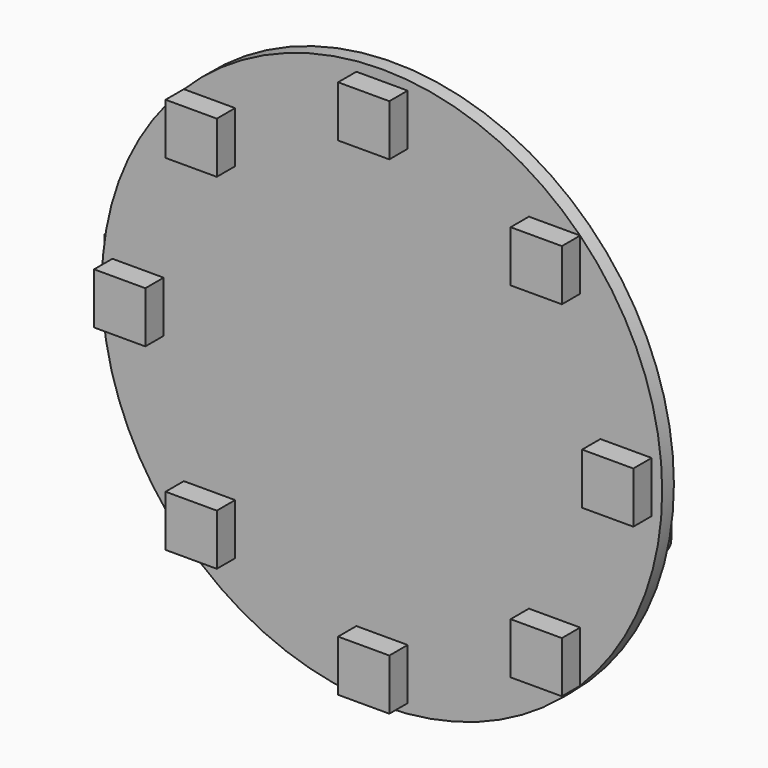
from build123d import *

# Parameters (mm, degrees)
F0_R      = 30.625
F1_DEPTH  = 1.6
F2_W      = 5.6
F2_H      = 5.6
F3_DEPTH  = 2.5
F4_W      = 16
F4_H      = 16
F5_DEPTH  = 1.6
F4_W_2    = 5.6
F4_H_2    = 5.6
F6_DEPTH  = 2.5
F4_W_3    = 3.4
F4_H_3    = 3
F4_W_4    = 1
F4_H_4    = 1.4143656492
F7_DEPTH  = 2.5
F8_DEPTH  = 3.5
F4_W_5    = 19
F4_H_5    = 8
F10_DEPTH = 4.5
F4_W_6    = 4.9
F4_H_6    = 11.6
F11_DEPTH = 0.7
F12_DEPTH = 4.3
F13_DEPTH = 3.5


# Not quite as in the source:
# - the program builds the solid bodies; features that only make, move or delete a surface that nothing else refers to are left out


with BuildPart() as f1:
    # F0 (on Front) → F1 (new body)
    with BuildSketch(Plane.XZ):
        Circle(F0_R)
    extrude(amount=F1_DEPTH)

    # F2 (on face) → F3 (join)
    with BuildSketch(Plane.XZ.offset(1.6)):
        with Locations((-26.67, 0)):
            Rectangle(F2_W, F2_H)
        with Locations((-18.8585378542, 18.8585378542)):
            Rectangle(F2_W, F2_H)
        with Locations((0, 26.67)):
            Rectangle(F2_W, F2_H)
        with Locations((18.8585378542, 18.8585378542)):
            Rectangle(F2_W, F2_H)
        with Locations((26.67, 0)):
            Rectangle(F2_W, F2_H)
        with Locations((18.8585378542, -18.8585378542)):
            Rectangle(F2_W, F2_H)
        with Locations((0, -26.67)):
            Rectangle(F2_W, F2_H)
        with Locations((-18.8585378542, -18.8585378542)):
            Rectangle(F2_W, F2_H)
    extrude(amount=F3_DEPTH)

    # F4 (on face) → F5 (join)
    with BuildSketch(Plane(origin=(0, 0, 0), x_dir=(-1, 0, 0), z_dir=(0, 1, 0))):
        with Locations((-9, -7)):
            Rectangle(F4_W, F4_H)
    extrude(amount=F5_DEPTH)

    # F4 (on face) → F6 (join)
    with BuildSketch(Plane(origin=(0, 0, 0), x_dir=(-1, 0, 0), z_dir=(0, 1, 0))):
        with Locations((0, 25)):
            Rectangle(F4_W_2, F4_H_2)
    extrude(amount=F6_DEPTH)

    # F4 (on face) → F7 (join)
    with BuildSketch(Plane(origin=(0, 0, 0), x_dir=(-1, 0, 0), z_dir=(0, 1, 0))):
        with Locations((7, 24)):
            Rectangle(F4_W_3, F4_H_3)
        with Locations((7, 24)):
            Rectangle(F4_W_4, F4_H_4, mode=Mode.SUBTRACT)
    extrude(amount=F7_DEPTH)

    # F4 (on face) → F8 (join)
    with BuildSketch(Plane(origin=(0, 0, 0), x_dir=(-1, 0, 0), z_dir=(0, 1, 0))):
        with Locations((7, 24)):
            Rectangle(F4_W_4, F4_H_4)
    extrude(amount=F8_DEPTH)

    # F4 (on face) → F10 (join)
    with BuildSketch(Plane(origin=(0, 0, 0), x_dir=(-1, 0, 0), z_dir=(0, 1, 0))):
        with Locations((0, -22.225)):
            Rectangle(F4_W_5, F4_H_5)
    extrude(amount=F10_DEPTH)

    # F4 (on face) → F11 (join)
    with BuildSketch(Plane(origin=(0, 0, 0), x_dir=(-1, 0, 0), z_dir=(0, 1, 0))):
        with Locations((-25, -5)):
            Rectangle(F4_W_6, F4_H_6)
        with BuildLine():
            ThreePointArc((-26.9, -1.75), (-25, 0.15), (-23.1, -1.75))
            Line((-23.1, -1.75), (-23.1, -8.25))
            ThreePointArc((-23.1, -8.25), (-25, -10.15), (-26.9, -8.25))
            Line((-26.9, -8.25), (-26.9, -1.75))
        make_face(mode=Mode.SUBTRACT)
    extrude(amount=F11_DEPTH)

    # F4 (on face) → F12 (join)
    with BuildSketch(Plane(origin=(0, 0, 0), x_dir=(-1, 0, 0), z_dir=(0, 1, 0))):
        with BuildLine():
            Line((-23.1, -8.25), (-23.1, -1.75))
            ThreePointArc((-23.1, -1.75), (-25, 0.15), (-26.9, -1.75))
            Line((-26.9, -1.75), (-26.9, -8.25))
            ThreePointArc((-26.9, -8.25), (-25, -10.15), (-23.1, -8.25))
        make_face()
    extrude(amount=F12_DEPTH)

    # F4 (on face) → F13 (join)
    with BuildSketch(Plane(origin=(0, 0, 0), x_dir=(-1, 0, 0), z_dir=(0, 1, 0))):
        with BuildLine():
            Line((24.005, -3.81), (30.387078257, -3.81))
            ThreePointArc((30.387078257, -3.81), (30.5654616898, -1.90871074), (30.625, 0))
            ThreePointArc((30.625, 0), (30.5654616898, 1.90871074), (30.387078257, 3.81))
            Line((30.387078257, 3.81), (24.005, 3.81))
            Line((24.005, 3.81), (24.005, -3.81))
        make_face()
        with BuildLine():
            Line((30.387078257, -3.81), (31.625, -3.81))
            Line((31.625, -3.81), (31.625, 3.81))
            Line((31.625, 3.81), (30.387078257, 3.81))
            ThreePointArc((30.387078257, 3.81), (30.5654616898, 1.90871074), (30.625, 0))
            ThreePointArc((30.625, 0), (30.5654616898, -1.90871074), (30.387078257, -3.81))
        make_face()
    extrude(amount=F13_DEPTH)


solid = f1.part
